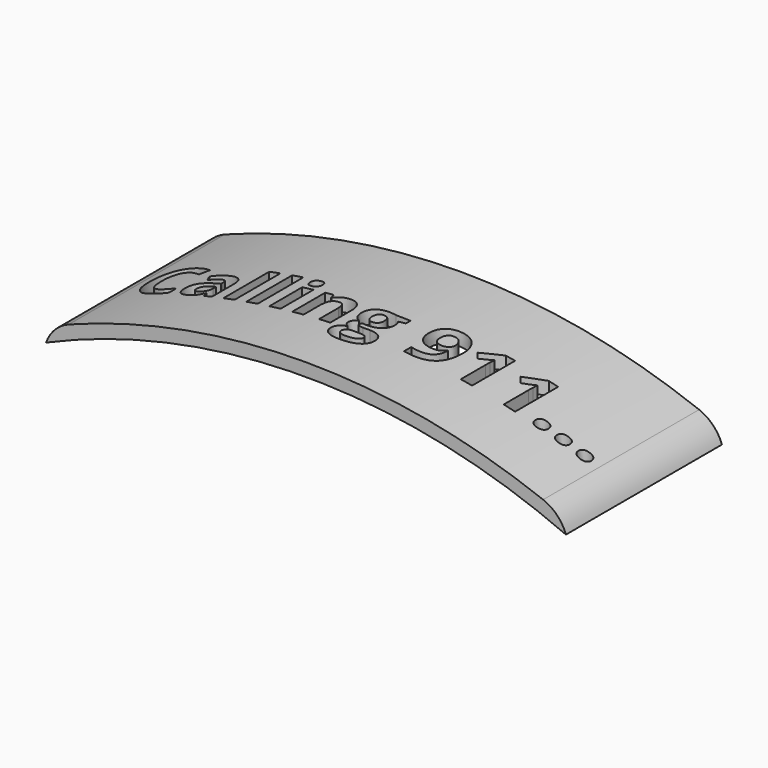
from build123d import *

# Parameters (mm, degrees)
F1_DEPTH     = 19.05
F3_TEXT_SIZE = 7.3573206608
F4_DEPTH     = 7.112
F5_T1_DEPTH  = 31.0660118863


# Not quite as in the source:
# - a fillet or chamfer that OpenCascade refuses, or shapes differently, is made with other operations: its cross-section is extruded or revolved along the edge and cut away or added
# - Text() gives the source's letters only with a copy of the font that has no kerning and outlines rounded to 1/6400 em; it was checked with that copy


with BuildPart() as f1:
    # F0 (on Front) → F1 (new body)
    with BuildSketch(Plane.XZ):
        with BuildLine():
            ThreePointArc((-25.4, 58.1987113259), (0, 63.5), (25.4, 58.1987113259))
            Line((25.4, 58.1987113259), (25.4, 59.5818168572))
            ThreePointArc((25.4, 59.5818168572), (0, 64.77), (-25.4, 59.5818168572))
            Line((-25.4, 59.5818168572), (-25.4, 58.1987113259))
        make_face()
    extrude(amount=F1_DEPTH)

    # F3 (on offset) → F4 (cut)
    with BuildSketch(Plane.XY.offset(66.04)):
        with Locations((-22.86, -12.7)):
            Text('Calling 911...', F3_TEXT_SIZE, font='Open Sans', font_style=FontStyle.BOLD, text_align=(TextAlign.LEFT, TextAlign.BOTTOM))
    extrude(amount=-F4_DEPTH, mode=Mode.SUBTRACT)

    # F5: fillet of radius 3.81 on 2 edges, made by hand

    # F5_s2 → F5_t1 (cut)
    with BuildSketch(Plane.XZ.offset(-6.0080059432)):
        with BuildLine():
            ThreePointArc((23.172194701, 60.4830744319), (24.5367559202, 59.5853454742), (25.4, 58.1987113259))
            Line((25.4, 58.1987113259), (25.4, 59.5818168572))
            ThreePointArc((25.4, 59.5818168572), (24.2902777016, 60.0427789928), (23.172194701, 60.4830744319))
        make_face()
        with BuildLine():
            ThreePointArc((-25.4, 58.1987113259), (-24.5367559202, 59.5853454742), (-23.172194701, 60.4830744319))
            ThreePointArc((-23.172194701, 60.4830744319), (-24.2902777016, 60.0427789928), (-25.4, 59.5818168572))
            Line((-25.4, 59.5818168572), (-25.4, 58.1987113259))
        make_face()
    extrude(amount=F5_T1_DEPTH, mode=Mode.SUBTRACT)


solid = f1.part
